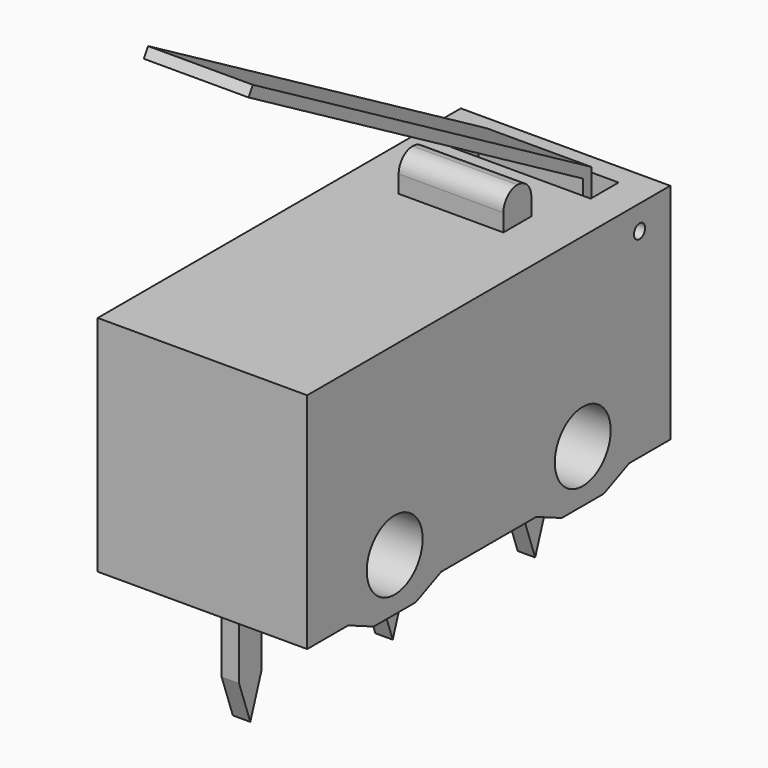
from build123d import *

# Parameters (mm, degrees)
F0_R      = 1
F0_R_2    = 0.2
F1_DEPTH  = 3
F3_DEPTH  = 0.25
F5_DEPTH  = 2
F6_DEPTH  = 1
F7_R      = 0.49999
F9_DEPTH  = 1.5
F10_DEPTH = 2.5


# Not quite as in the source:
# - a fillet or chamfer is up to 0.001 mm smaller than in the source, because OpenCascade refuses the exact size


with BuildPart() as f1:
    # F0 (on Right) → F1 (new body, symmetric)
    with BuildSketch(Plane.YZ):
        Polygon((0, 3.2), (-6.5, 3.2), (-6.5, -3.2), (-5.033030278, -3.2), (-4.116515139, -3.6), (-2.616515139, -3.6), (-1.7, -3.2), (0, -3.2), (1.7, -3.2), (2.616515139, -3.6), (4.116515139, -3.6), (5.033030278, -3.2), (6.5, -3.2), (6.5, 3.2), align=None)
        with Locations((-3.366515139, -2.1)):
            Circle(F0_R, mode=Mode.SUBTRACT)
        with Locations((3.366515139, -2.1)):
            Circle(F0_R, mode=Mode.SUBTRACT)
        with Locations((5.4, 2.5)):
            Circle(F0_R_2, mode=Mode.SUBTRACT)
    extrude(amount=F1_DEPTH, both=True)

    # F2 (on Right) → F3 (join, symmetric)
    with BuildSketch(Plane.YZ):
        Polygon((-4.7, -3.2), (-5.5, -3.2), (-5.5, -5.3686291501), (-5.1, -6.5), (-4.7, -5.3686291501), align=None)
        Polygon((0, -6.5), (0.4, -5.3686291501), (0.4, -3.2), (-0.4, -3.2), (-0.4, -5.3686291501), align=None)
        Polygon((5.1, -6.5), (5.5, -5.3686291501), (5.5, -3.2), (4.7, -3.2), (4.7, -5.3686291501), align=None)
    extrude(amount=F3_DEPTH, both=True)

    # F4 (on face) → F5 (cut)
    with BuildSketch(Plane.XY.offset(3.2)):
        Polygon((2, 5.9), (0, 5.9), (-2, 5.9), (-2, 4.9), (0, 4.9), (2, 4.9), align=None)
    extrude(amount=-F5_DEPTH, mode=Mode.SUBTRACT)

    # F4 (on face) → F6 (join)
    with BuildSketch(Plane.XY.offset(3.2)):
        Polygon((1.5, 3.4), (0, 3.4), (-1.5, 3.4), (-1.5, 2.4), (0, 2.4), (1.5, 2.4), align=None)
    extrude(amount=F6_DEPTH)

    # F7 (radius 0.5 in the source; OpenCascade refuses exactly that, so slightly less here)
    f7_edges = [f1.edges().sort_by_distance(p)[0] for p in [
        (0, 3.4, 4.2),
        (0, 2.4, 4.2),
    ]]
    fillet(f7_edges, radius=F7_R)


with BuildPart() as f9:
    # F8 (on Right) → F9 (new body, symmetric)
    with BuildSketch(Plane.YZ):
        with BuildLine():
            ThreePointArc((5.25, 2.5), (5.4, 2.65), (5.55, 2.5))
            Line((5.55, 2.5), (5.55, 3.5732050808))
            Line((5.55, 3.5732050808), (-6.574355653, 10.5732050808))
            Line((-6.574355653, 10.5732050808), (-6.724355653, 10.3133974596))
            Line((-6.724355653, 10.3133974596), (5.25, 3.4))
            Line((5.25, 3.4), (5.25, 2.5))
        make_face()
    extrude(amount=F9_DEPTH, both=True)

    # F8 (on Right) → F10 (join, symmetric)
    with BuildSketch(Plane.YZ):
        with BuildLine():
            ThreePointArc((5.25, 2.5), (5.4, 2.35), (5.55, 2.5))
            ThreePointArc((5.55, 2.5), (5.4, 2.65), (5.25, 2.5))
        make_face()
    extrude(amount=F10_DEPTH, both=True)


solid = Compound([f1.part, f9.part])
